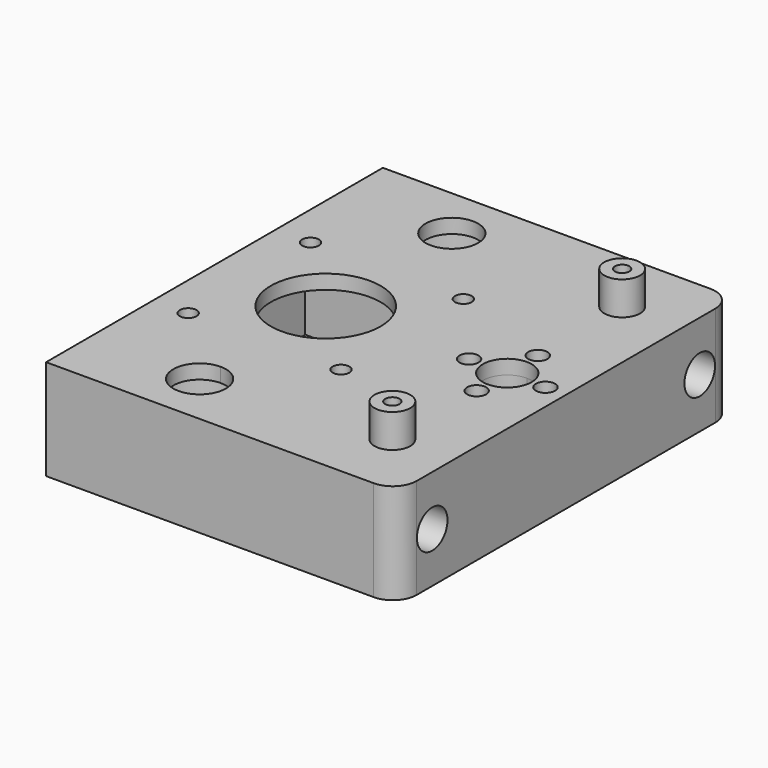
from build123d import *

# Parameters (mm, degrees)
F1_DEPTH  = 2
F2_R      = 9.75
F2_W      = 43
F2_H      = 43
F2_R_2    = 11.25
F2_R_3    = 2
F3_DEPTH  = 16
F4_R      = 9.75
F4_R_2    = 2
F4_W      = 43
F4_H      = 43
F4_R_3    = 5.1
F4_R_4    = 1.75
F4_R_5    = 11.5
F5_DEPTH  = 3
F7_DEPTH  = 40
F6_R      = 4
F8_DEPTH  = 35
F9_R      = 3.75
F9_R_2    = 1.5
F10_DEPTH = 7


# Not quite as in the source:
# - after a boolean that leaves OpenCascade's solid faulty, fix() repairs it
# - a feature names something its author has since deleted; it is built from what else it names


with BuildPart() as f1:
    # F0 (on Top) → F1 (new body)
    with BuildSketch(Plane.XY):
        with BuildLine():
            Line((45.2909459174, 44.0599285066), (23.2912804931, 44.0599285066))
            Line((23.2912804931, 44.0599285066), (-23.2912804931, 44.0599285066))
            Line((-23.2912804931, 44.0599285066), (-23.2912804931, -44.0599285066))
            Line((-23.2912804931, -44.0599285066), (23.2912804931, -44.0599285066))
            Line((23.2912804931, -44.0599285066), (45.2909459174, -44.0599285066))
            ThreePointArc((45.2909459174, -44.0599285066), (48.8264798233, -42.5954624125), (50.2909459174, -39.0599285066))
            Line((50.2909459174, -39.0599285066), (50.2909459174, -23.5600714934))
            Line((50.2909459174, -23.5600714934), (50.2909459174, 23.5599285066))
            Line((50.2909459174, 23.5599285066), (50.2909459174, 39.0599285066))
            ThreePointArc((50.2909459174, 39.0599285066), (48.8264798233, 42.5954624125), (45.2909459174, 44.0599285066))
        make_face()
        with BuildLine():
            ThreePointArc((9.75, -33), (-6.8942911166, -39.8942911166), (0, -23.25))
            ThreePointArc((0, -23.25), (6.8942911166, -26.1057088834), (9.75, -33))
        make_face(mode=Mode.SUBTRACT)
        Polygon((21.5, 21.5), (21.5, 0), (21.5, -21.5), (0, -21.5), (-21.5, -21.5), (-21.5, 21.5), (0, 21.5), (21.4772019535, 21.5), align=None, mode=Mode.SUBTRACT)
        with BuildLine():
            ThreePointArc((9.75, 33), (6.8942911166, 26.1057088834), (0, 23.25))
            ThreePointArc((0, 23.25), (-6.8942911166, 39.8942911166), (9.75, 33))
        make_face(mode=Mode.SUBTRACT)
        with BuildLine():
            ThreePointArc((26.75, 0), (38, 11.25), (49.25, 0))
            ThreePointArc((49.25, 0), (38, -11.25), (26.75, 0))
        make_face(mode=Mode.SUBTRACT)
    extrude(amount=F1_DEPTH)

    # F2 (on face) → F3 (join)
    with BuildSketch(Plane.XY.offset(2)):
        with BuildLine():
            ThreePointArc((50.2909459174, 39.0599285066), (48.8264798233, 42.5954624125), (45.2909459174, 44.0599285066))
            Line((45.2909459174, 44.0599285066), (-23.2912804931, 44.0599285066))
            Line((-23.2912804931, 44.0599285066), (-23.2912804931, -44.0599285066))
            Line((-23.2912804931, -44.0599285066), (45.2909459174, -44.0599285066))
            ThreePointArc((45.2909459174, -44.0599285066), (48.8264798233, -42.5954624125), (50.2909459174, -39.0599285066))
            Line((50.2909459174, -39.0599285066), (50.2909459174, 39.0599285066))
        make_face()
        with Locations((0, -33)):
            Circle(F2_R, mode=Mode.SUBTRACT)
        Rectangle(F2_W, F2_H, mode=Mode.SUBTRACT)
        with Locations((0, 33)):
            Circle(F2_R, mode=Mode.SUBTRACT)
        with Locations((38, 0)):
            Circle(F2_R_2, mode=Mode.SUBTRACT)
        with Locations((38, 0)):
            Circle(F2_R_2)
        with Locations((38, -8)):
            Circle(F2_R_3, mode=Mode.SUBTRACT)
        with Locations((30, 0)):
            Circle(F2_R_3, mode=Mode.SUBTRACT)
        with BuildLine():
            ThreePointArc((38, 5.1), (41.6062445841, 3.6062445841), (43.1, 0))
            ThreePointArc((43.1, 0), (34.3937554159, -3.6062445841), (38, 5.1))
        make_face(mode=Mode.SUBTRACT)
        with BuildLine():
            ThreePointArc((40, 8), (39.4142135624, 6.5857864376), (38, 6))
            ThreePointArc((38, 6), (36.5857864376, 9.4142135624), (40, 8))
        make_face(mode=Mode.SUBTRACT)
        with BuildLine():
            ThreePointArc((48, 0), (46, -2), (44, 0))
            ThreePointArc((44, 0), (46, 2), (48, 0))
        make_face(mode=Mode.SUBTRACT)
    extrude(amount=F3_DEPTH)

    # F4 (on face) → F5 (join)
    with BuildSketch(Plane.XY.offset(18)):
        with BuildLine():
            Line((50.2909459174, -39.0599285066), (50.2909459174, 39.0599285066))
            ThreePointArc((50.2909459174, 39.0599285066), (48.8264798233, 42.5954624125), (45.2909459174, 44.0599285066))
            Line((45.2909459174, 44.0599285066), (-23.2912804931, 44.0599285066))
            Line((-23.2912804931, 44.0599285066), (-23.2912804931, -44.0599285066))
            Line((-23.2912804931, -44.0599285066), (45.2909459174, -44.0599285066))
            ThreePointArc((45.2909459174, -44.0599285066), (48.8264798233, -42.5954624125), (50.2909459174, -39.0599285066))
        make_face()
        with Locations((0, -33)):
            Circle(F4_R, mode=Mode.SUBTRACT)
        with Locations((38, -8)):
            Circle(F4_R_2, mode=Mode.SUBTRACT)
        Rectangle(F4_W, F4_H, mode=Mode.SUBTRACT)
        with Locations((0, 33)):
            Circle(F4_R, mode=Mode.SUBTRACT)
        with Locations((30, 0)):
            Circle(F4_R_2, mode=Mode.SUBTRACT)
        with Locations((38, 0)):
            Circle(F4_R_3, mode=Mode.SUBTRACT)
        with Locations((38, 8)):
            Circle(F4_R_2, mode=Mode.SUBTRACT)
        with Locations((46, 0)):
            Circle(F4_R_2, mode=Mode.SUBTRACT)
        Rectangle(F4_W, F4_H)
        with Locations((-16, -16)):
            Circle(F4_R_4, mode=Mode.SUBTRACT)
        with Locations((16, -16)):
            Circle(F4_R_4, mode=Mode.SUBTRACT)
        with Locations((-16, 16)):
            Circle(F4_R_4, mode=Mode.SUBTRACT)
        Circle(F4_R_5, mode=Mode.SUBTRACT)
        with Locations((16, 16)):
            Circle(F4_R_4, mode=Mode.SUBTRACT)
        with Locations((0, -33)):
            Circle(F4_R)
        with Locations((0, 33)):
            Circle(F4_R)
    extrude(amount=F5_DEPTH)

    # F0 (on Top) → F7 (cut)
    with BuildSketch(Plane.XY):
        with BuildLine():
            ThreePointArc((5.5, -33), (3.8890872965, -29.1109127035), (0, -27.5))
            ThreePointArc((0, -27.5), (-3.8890872965, -36.8890872965), (5.5, -33))
        make_face()
        with BuildLine():
            ThreePointArc((5.5, 33), (-3.8890872965, 36.8890872965), (0, 27.5))
            ThreePointArc((0, 27.5), (3.8890872965, 29.1109127035), (5.5, 33))
        make_face()
    extrude(amount=F7_DEPTH, mode=Mode.SUBTRACT)

    add(f1.part.fix(), mode=Mode.REPLACE)

    # F6 (on face) → F8 (cut)
    with BuildSketch(Plane.YZ.offset(50.2909459174)):
        with Locations((35, 10.5)):
            Circle(F6_R)
        with Locations((-35, 10.5)):
            Circle(F6_R)
    extrude(amount=-F8_DEPTH, mode=Mode.SUBTRACT)

    # F9 (on face) → F10 (join)
    with BuildSketch(Plane.XY.offset(21)):
        with Locations((37.9999959174, 30.0599285066)):
            Circle(F9_R)
        with Locations((37.9999959174, 30.0599285066)):
            Circle(F9_R_2, mode=Mode.SUBTRACT)
        with Locations((37.9999959174, -30.0599285066)):
            Circle(F9_R)
        with Locations((37.9999959174, -30.0599285066)):
            Circle(F9_R_2, mode=Mode.SUBTRACT)
    extrude(amount=F10_DEPTH)


solid = f1.part
